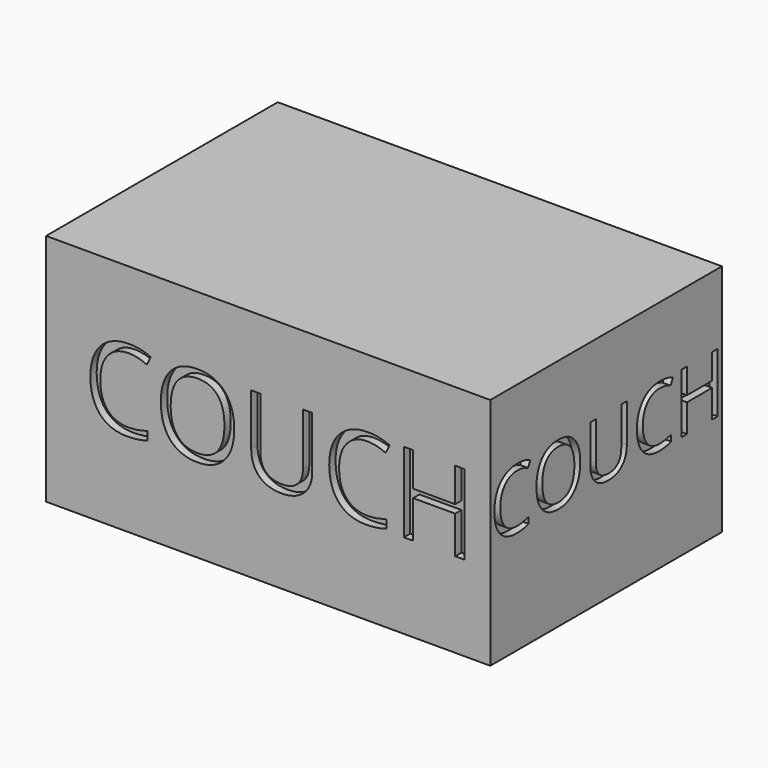
from build123d import *

# Parameters (mm, degrees)
F0_W         = 1422.4
F0_H         = 749.3
F1_DEPTH     = 463.55
F2_TEXT_SIZE = 357.810407877
F3_DEPTH     = 25.4
F4_TEXT_SIZE = 266.899374747
F5_DEPTH     = 25.4


# Not quite as in the source:
# - Text() gives the source's letters only with a copy of the font that has no kerning and outlines rounded to 1/6400 em; it was checked with that copy


with BuildPart() as f1:
    # F0 (on Front) → F1 (new body, symmetric)
    with BuildSketch(Plane.XZ):
        Rectangle(F0_W, F0_H)
    extrude(amount=F1_DEPTH, both=True)

    # F2 (on face) → F3 (cut)
    with BuildSketch(Plane.XZ.offset(463.55)):
        with Locations((-591.3030207157, -102.4772971869)):
            Text('COUCH', F2_TEXT_SIZE, font='Open Sans', text_align=(TextAlign.LEFT, TextAlign.BOTTOM))
    extrude(amount=-F3_DEPTH, mode=Mode.SUBTRACT)

    # F4 (on face) → F5 (cut)
    with BuildSketch(Plane.YZ.offset(711.2)):
        with Locations((-463.55, -41.5027735926)):
            Text('COUCH', F4_TEXT_SIZE, font='Open Sans', text_align=(TextAlign.LEFT, TextAlign.BOTTOM))
    extrude(amount=-F5_DEPTH, mode=Mode.SUBTRACT)


solid = f1.part
